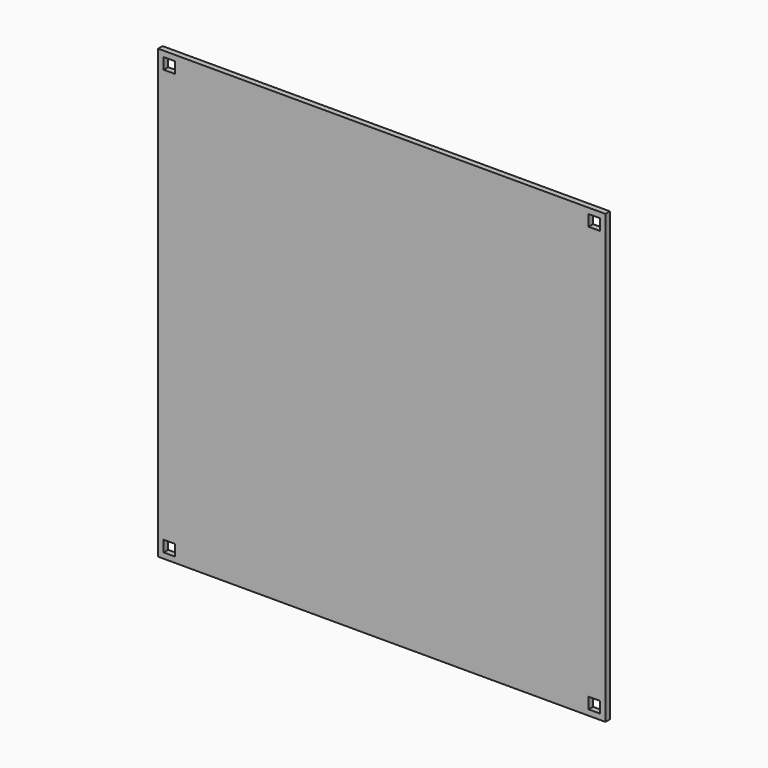
from build123d import *

# Parameters (mm, degrees)
F1_W     = 240
F1_H     = 240
F1_W_2   = 6
F1_H_2   = 6
F2_DEPTH = 3
F3_DEPTH = 25


with BuildPart() as f2:
    # F1 (on Front) → F2 (new body)
    with BuildSketch(Plane.XZ):
        with Locations((120, 120)):
            Rectangle(F1_W, F1_H)
        with Locations((6, 234)):
            Rectangle(F1_W_2, F1_H_2, mode=Mode.SUBTRACT)
        with Locations((6, 234)):
            Rectangle(F1_W_2, F1_H_2)
    extrude(amount=F2_DEPTH)

    # F1 (on Front) → F3 (cut)
    with BuildSketch(Plane.XZ):
        with Locations((6, 234)):
            Rectangle(F1_W_2, F1_H_2)
    extrude(amount=F3_DEPTH, mode=Mode.SUBTRACT)

    # F5: F2 across plane


with BuildPart() as f2_1:
    add(f2.part)
    add(f2.part.mirror(Plane(origin=(120, -1.5, 120), x_dir=(0, -1, 0), z_dir=(-1, 0, 0))), mode=Mode.INTERSECT)

    # F7: F2 across plane


with BuildPart() as f2_2:
    add(f2_1.part)
    add(f2_1.part.mirror(Plane(origin=(120, -1.5, 120), x_dir=(1, 0, 0), z_dir=(0, 0, 1))), mode=Mode.INTERSECT)


solid = f2_2.part
